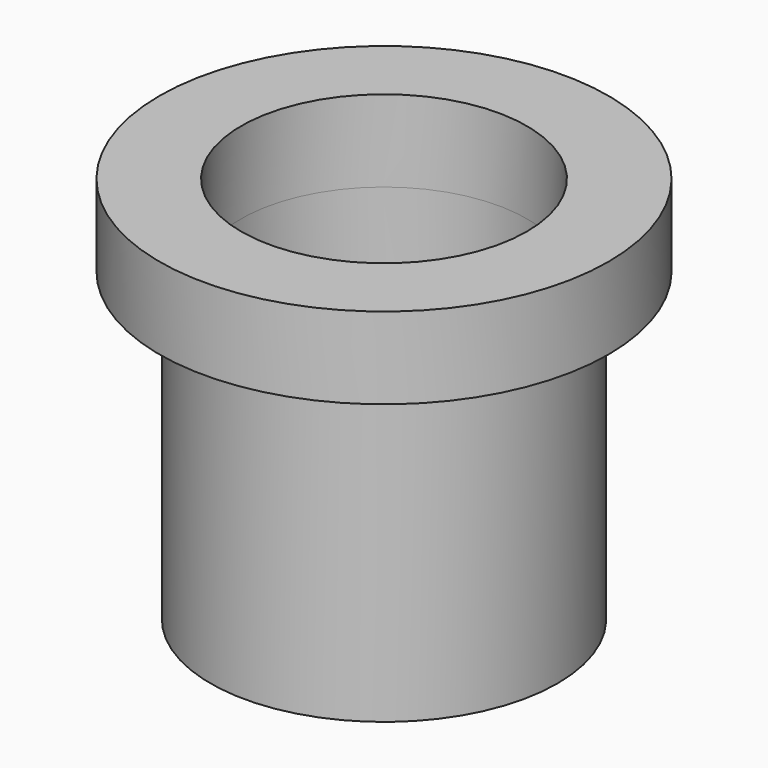
from build123d import *

# Parameters (mm, degrees)
F0_R     = 5.5
F0_R_2   = 4.25
F0_R_3   = 3.5
F1_DEPTH = 2
F2_DEPTH = 7.5


# Not quite as in the source:
# - a feature names something its author has since deleted; it is built from what else it names


with BuildPart() as f1:
    # F0 (on Top) → F1 (new body)
    with BuildSketch(Plane.XY):
        Circle(F0_R)
        Circle(F0_R_2, mode=Mode.SUBTRACT)
        Circle(F0_R_2)
        Circle(F0_R_3, mode=Mode.SUBTRACT)
    extrude(amount=F1_DEPTH)

    # F0 (on Top) → F2 (join)
    with BuildSketch(Plane.XY):
        Circle(F0_R_2)
        Circle(F0_R_3, mode=Mode.SUBTRACT)
    extrude(amount=-F2_DEPTH)


solid = f1.part
